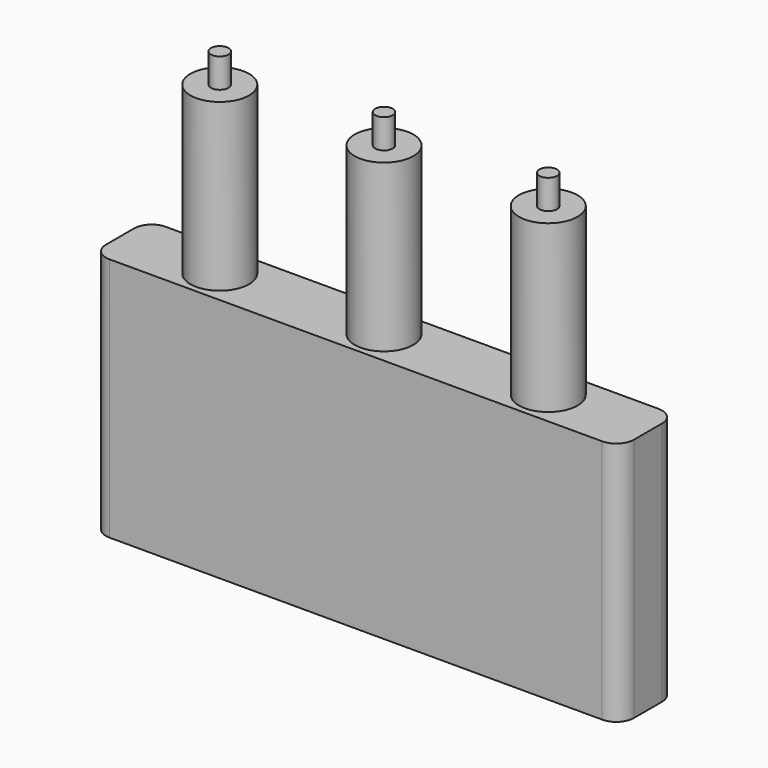
from build123d import *

# Parameters (mm, degrees)
F0_W     = 90
F0_H     = 41.77
F1_DEPTH = 6
F3_DEPTH = 28.33
F4_R     = 3
F5_R     = 1.5
F6_DEPTH = 5


with BuildPart() as f1:
    # F0 (on Front) → F1 (new body, symmetric)
    with BuildSketch(Plane.XZ):
        Rectangle(F0_W, F0_H)
    extrude(amount=F1_DEPTH, both=True)

    # F2 (on face) → F3 (join)
    with BuildSketch(Plane.XY.offset(20.885)):
        with BuildLine():
            Line((-28, 0), (-23, 0))
            ThreePointArc((-23, 0), (-28, 5), (-33, 0))
            Line((-33, 0), (-28, 0))
        make_face()
        with BuildLine():
            ThreePointArc((-33, 0), (-28, -5), (-23, 0))
            Line((-23, 0), (-28, 0))
            Line((-28, 0), (-33, 0))
        make_face()
        with BuildLine():
            Line((-5, 0), (0, 0))
            Line((0, 0), (5, 0))
            ThreePointArc((5, 0), (0, 5), (-5, 0))
        make_face()
        with BuildLine():
            Line((5, 0), (0, 0))
            Line((0, 0), (-5, 0))
            ThreePointArc((-5, 0), (0, -5), (5, 0))
        make_face()
        with BuildLine():
            ThreePointArc((33, 0), (28, 5), (23, 0))
            ThreePointArc((23, 0), (28, -5), (33, 0))
        make_face()
    extrude(amount=F3_DEPTH)

    # F4
    f4_edges = [f1.edges().sort_by_distance(p)[0] for p in [
        (45, -6, 0),
        (45, 6, 0),
        (-45, -6, 0),
        (-45, 6, 0),
    ]]
    fillet(f4_edges, radius=F4_R)

    # F5 (on face) → F6 (join)
    with BuildSketch(Plane.XY.offset(49.215)):
        with Locations((-28, 0)):
            Circle(F5_R)
        Circle(F5_R)
        with Locations((28, 0)):
            Circle(F5_R)
    extrude(amount=F6_DEPTH)


solid = f1.part
